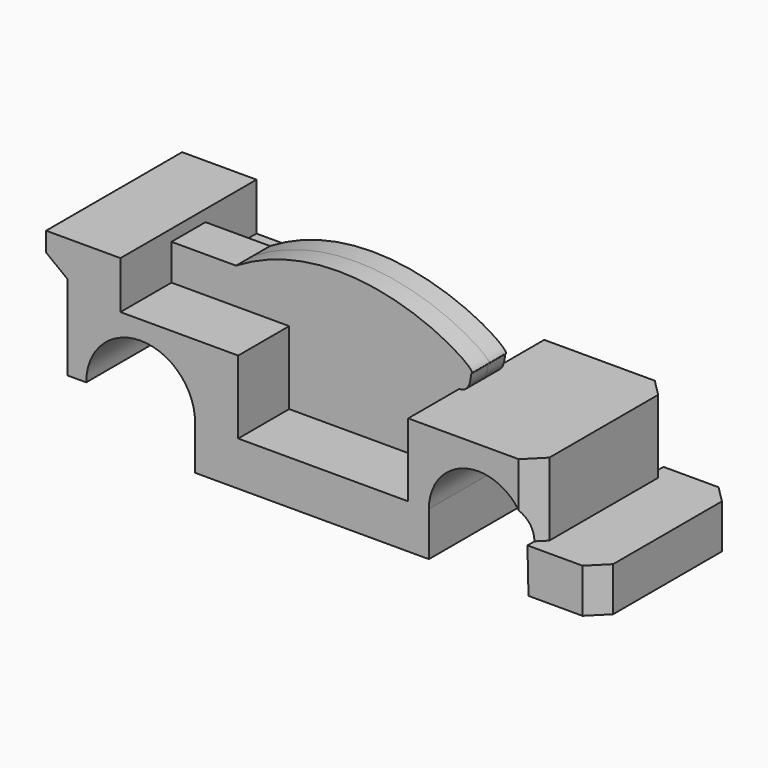
from build123d import *

# Parameters (mm, degrees)
F1_DEPTH    = 25.4
F0_W        = 19.2914952449
F0_H        = 10.7399431888
F2_DEPTH    = 6.35
F0_W_2      = 50.8
F0_H_2      = 21.8239631504
F3_DEPTH    = 6.35
F4_DEPTH    = 25.4
F5_DEPTH    = 6.35
F7_DEPTH    = 25.4
F8_SIZE     = 5.08
F9_T1_DEPTH = 34.8881127292


# Not quite as in the source:
# - a fillet or chamfer that OpenCascade refuses, or shapes differently, is made with other operations: its cross-section is extruded or revolved along the edge and cut away or added


with BuildPart() as f1:
    # F0 (on Front) → F1 (new body, symmetric)
    with BuildSketch(Plane.XZ):
        with BuildLine():
            Line((-75.1296169648, 36.0071417369), (-97.3546169648, 36.0071417369))
            Line((-97.3546169648, 36.0071417369), (-97.3546169648, 30.2704927005))
            Line((-97.3546169648, 30.2704927005), (-91.0229831883, 25.4))
            Line((-91.0229831883, 25.4), (-91.0229831883, 0))
            Line((-91.0229831883, 0), (-85.3649152333, 0))
            ThreePointArc((-85.3649152333, 0), (-69.097654886, 16.2672603473), (-52.8303945387, 0))
            Line((-52.8303945387, 0), (-39.9631213073, 0))
            Line((-39.9631213073, 0), (-39.9631213073, 21.8239631504))
            Line((-39.9631213073, 21.8239631504), (-55.8381217199, 21.8239631504))
            Line((-55.8381217199, 21.8239631504), (-75.1296169648, 21.8239631504))
            Line((-75.1296169648, 21.8239631504), (-75.1296169648, 32.5639063391))
            Line((-75.1296169648, 32.5639063391), (-75.1296169648, 36.0071417369))
        make_face()
    extrude(amount=F1_DEPTH, both=True)

    # F0 (on Front) → F2 (join, symmetric)
    with BuildSketch(Plane.XZ):
        with Locations((-65.4838693423, 27.1939347448)):
            Rectangle(F0_W, F0_H)
    extrude(amount=F2_DEPTH, both=True)

    # F0 (on Front) → F3 (join, symmetric)
    with BuildSketch(Plane.XZ):
        with Locations((-14.5631213073, 10.9119815752)):
            Rectangle(F0_W_2, F0_H_2)
    extrude(amount=F3_DEPTH, both=True)

    # F0 (on Front) → F4 (join, symmetric)
    with BuildSketch(Plane.XZ):
        with BuildLine():
            Line((-39.9631213073, 0), (-52.8303945387, 0))
            Line((-52.8303945387, 0), (-52.8303945387, -13.2021475583))
            Line((-52.8303945387, -13.2021475583), (17.0196054613, -13.2021475583))
            Line((17.0196054613, -13.2021475583), (17.0196054613, 0))
            ThreePointArc((17.0196054613, 0), (31.740901159, 14.7212956977), (46.4621968567, 0))
            Line((46.4621968567, 0), (48.9368786927, 0))
            Line((48.9368786927, 0), (48.9368786927, 21.8239631504))
            Line((48.9368786927, 21.8239631504), (10.8368786927, 21.8239631504))
            Line((10.8368786927, 21.8239631504), (10.8368786927, 0))
            Line((10.8368786927, 0), (-39.9631213073, 0))
        make_face()
    extrude(amount=F4_DEPTH, both=True)

    # F0 (on Front) → F5 (join, symmetric)
    with BuildSketch(Plane.XZ):
        with BuildLine():
            add(Edge.make_bspline(
                [(-55.8381217199, 32.5639063391), (-21.9943716528, 53.0867397368), (14.9422549228, 30.0580051652), (14.6605303397, 27.2929135664), (14.6510890776, 27.2561161473)],
                knots=[0, 0, 0, 0, 0.9196914564, 0.9333237743, 0.9333237743, 0.9333237743, 0.9333237743], degree=3))
            Line((-55.8381217199, 32.5639063391), (-55.8381217199, 21.8239631504))
            Line((-55.8381217199, 21.8239631504), (-39.9631213073, 21.8239631504))
            Line((-39.9631213073, 21.8239631504), (10.8368786927, 21.8239631504))
            add(Edge.make_bspline(
                [(10.8368786927, 21.8239631504), (14.3414601512, 21.8239631504), (14.1556344602, 26.013278758), (14.4361378277, 26.8880673131)],
                knots=[0, 0, 0, 0, 0.7087903715, 0.7087903715, 0.7087903715, 0.7087903715], degree=3))
            add(Edge.make_bspline(
                [(14.4670024546, 26.9684424726), (14.4472838381, 26.9404074645), (14.4347952429, 26.9142327885), (14.4361378277, 26.8880673131)],
                knots=[0.9814355703, 0.9814355703, 0.9814355703, 0.9814355703, 1, 1, 1, 1], degree=3))
            add(Edge.make_bspline(
                [(14.4670024546, 26.9684424726), (14.521048149, 27.0861460429), (14.5831737171, 27.1208715793), (14.6206044517, 27.1763895775)],
                knots=[0.7335614759, 0.7335614759, 0.7335614759, 0.7335614759, 0.8588119226, 0.8588119226, 0.8588119226, 0.8588119226], degree=3))
            add(Edge.make_bspline(
                [(14.6510890776, 27.2561161473), (14.6437422584, 27.2274818417), (14.6331701617, 27.2010214483), (14.6206044517, 27.1763895775)],
                knots=[0.9333237743, 0.9333237743, 0.9333237743, 0.9333237743, 0.9439319084, 0.9439319084, 0.9439319084, 0.9439319084], degree=3))
        make_face()
    extrude(amount=F5_DEPTH, both=True)

    # F0 (on Front) → F7 (join, symmetric)
    with BuildSketch(Plane.XZ):
        Polygon((48.9368786927, -13.1861399859), (48.9368786927, 0), (46.4621968567, 0), (46.7710867524, -13.1861399859), align=None)
        Polygon((59.2892281711, 0), (48.9368786927, 0), (48.9368786927, -13.1861399859), (67.9868786927, -13.1861399859), (67.9868786927, 0), align=None)
    extrude(amount=F7_DEPTH, both=True)

    # F8
    f8_edges = [f1.edges().sort_by_distance(p)[0] for p in [
        (67.986879, -25.4, -6.59307),
        (67.986879, 25.4, -6.59307),
    ]]
    chamfer(f8_edges, length=F8_SIZE)

    # F9: chamfer of 5.08 on 2 edges, made by hand

    # F9_s2 → F9_t1 (cut)
    with BuildSketch(Plane.XY):
        Polygon((48.9368786927, -20.32), (43.8568786927, -25.4), (48.9368786927, -25.4), align=None)
        Polygon((43.8568786927, 25.4), (48.9368786927, 20.32), (48.9368786927, 25.4), align=None)
    extrude(amount=F9_T1_DEPTH, mode=Mode.SUBTRACT)


solid = f1.part
